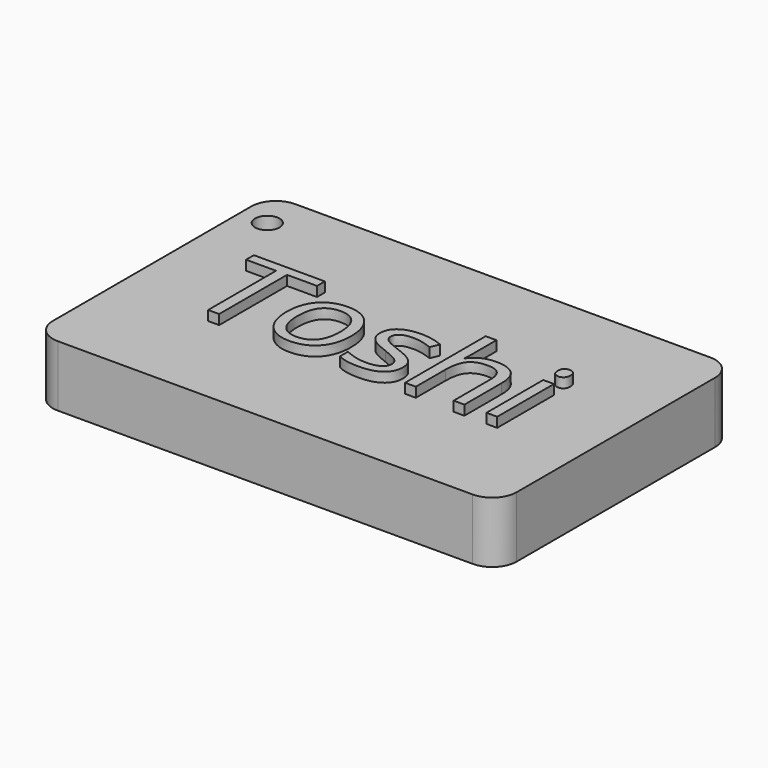
from build123d import *

# Parameters (mm, degrees)
F0_W         = 96.3954925537
F0_H         = 61.7070589215
F1_DEPTH     = 12.7
F2_TEXT_SIZE = 27.55490067
F3_DEPTH     = 2.032
F5_D         = 5.08
F7_R         = 5.08
F8_R         = 5.08


# Not quite as in the source:
# - Text() gives the source's letters only with a copy of the font that has no kerning and outlines rounded to 1/6400 em; it was checked with that copy


with BuildPart() as f1:
    # F0 (on Top) → F1 (new body)
    with BuildSketch(Plane.XY):
        with Locations((0.9587258101, -0.5229404196)):
            Rectangle(F0_W, F0_H)
    extrude(amount=F1_DEPTH)

    # F2 (on face) → F3 (join)
    with BuildSketch(Plane.XY.offset(12.7)):
        with Locations((-33.9950937778, -10.6049054302)):
            Text('Toshi', F2_TEXT_SIZE, font='Open Sans', text_align=(TextAlign.LEFT, TextAlign.BOTTOM))
    extrude(amount=F3_DEPTH)

    # F5 (through all)
    with Locations(Plane.XY.offset(12.7)):
        with Locations((-41.5671691298, 22.313028574)):
            Hole(F5_D / 2)

    # F7
    f7_edges = [f1.edges().sort_by_distance(p)[0] for p in [
        (-47.23902, -31.37647, 6.35),
    ]]
    fillet(f7_edges, radius=F7_R)

    # F8
    f8_edges = [f1.edges().sort_by_distance(p)[0] for p in [
        (-47.23902, 30.330589, 6.35),
        (-47.23902, -26.29647, 6.35),
        (49.156472, 30.330589, 6.35),
        (49.156472, -31.37647, 6.35),
    ]]
    fillet(f8_edges, radius=F8_R)


solid = f1.part
